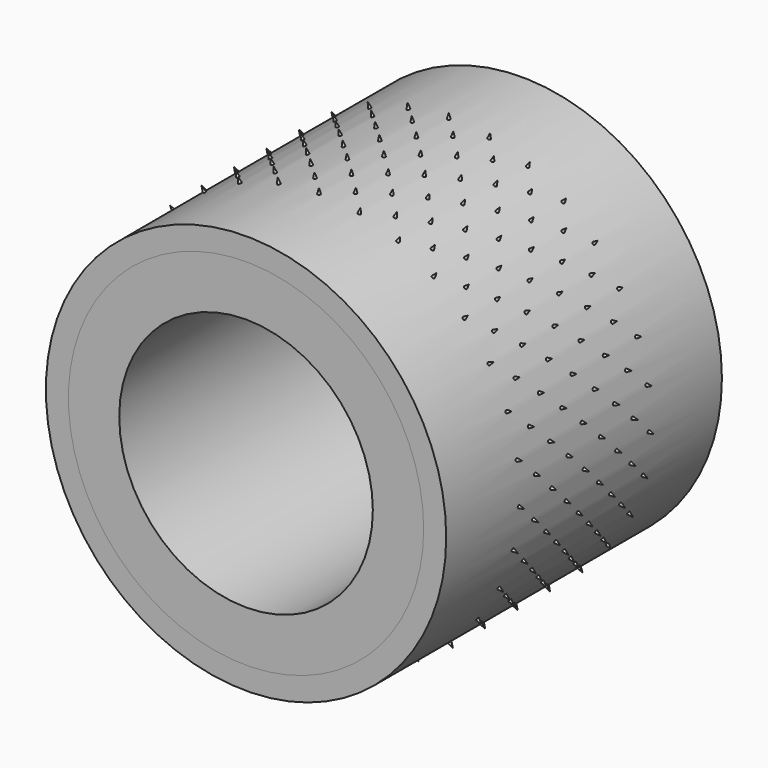
from build123d import *

# Parameters (mm, degrees)
F0_R        = 35.052
F0_R_2      = 25.019
F1_DEPTH    = 34
F2_R        = 39.5
F2_R_2      = 35.052
F3_DEPTH    = 34
F5_R        = 0.31
F6_DEPTH    = 25.4
F8_DEPTH    = 5.5
F9_SIZE2    = 0.31
F9_SIZE     = 1.1
F9_2_SIZE2  = 0.31
F9_2_SIZE   = 1.1
F9_3_SIZE2  = 0.31
F9_3_SIZE   = 1.1
F9_4_SIZE2  = 0.31
F9_4_SIZE   = 1.1
F9_5_SIZE2  = 0.31
F9_5_SIZE   = 1.1
F11_R       = 0.31
F12_DEPTH   = 25.4
F13_DEPTH   = 5.5
F14_SIZE2   = 0.31
F14_SIZE    = 1.1
F14_2_SIZE2 = 0.31
F14_2_SIZE  = 1.1
F14_3_SIZE2 = 0.31
F14_3_SIZE  = 1.1
F14_4_SIZE2 = 0.31
F14_4_SIZE  = 1.1
F15_COUNT   = 31
F15_ANGLE   = 348.387


with BuildPart() as f1:
    # F0 (on Front) → F1 (new body, symmetric)
    with BuildSketch(Plane.XZ):
        Circle(F0_R)
        Circle(F0_R_2, mode=Mode.SUBTRACT)
    extrude(amount=F1_DEPTH, both=True)


with BuildPart() as f3:
    # F2 (on Front) → F3 (new body, symmetric)
    with BuildSketch(Plane.XZ):
        Circle(F2_R)
        Circle(F2_R_2, mode=Mode.SUBTRACT)
    extrude(amount=F3_DEPTH, both=True)

    # F5 (on offset) → F6 (cut)
    with BuildSketch(Plane.XY.offset(35.052)):
        with Locations((0, -16)):
            Circle(F5_R)
        with Locations((0, -8)):
            Circle(F5_R)
        Circle(F5_R)
        with Locations((0, 16)):
            Circle(F5_R)
        with Locations((0, 8)):
            Circle(F5_R)
    extrude(amount=F6_DEPTH, mode=Mode.SUBTRACT)

    # F11 (on offset) → F12 (cut)
    with BuildSketch(Plane.XY.offset(-35.052)):
        with Locations((0, -4)):
            Circle(F11_R)
        with Locations((0, -12)):
            Circle(F11_R)
        with Locations((0, 12)):
            Circle(F11_R)
        with Locations((0, 4)):
            Circle(F11_R)
    extrude(amount=-F12_DEPTH, mode=Mode.SUBTRACT)


with BuildPart() as f8:
    # F5 (on offset) → F8 (new body)
    with BuildSketch(Plane.XY.offset(35.052)):
        with Locations((0, 16)):
            Circle(F5_R)
    extrude(amount=F8_DEPTH)

    # F9
    f9_edges = [f8.edges().sort_by_distance(p)[0] for p in [
        (-0.31, 16, 40.552),
    ]]
    f9_side = f8.faces().sort_by_distance((-0.31, 16, 37.802))[0]
    chamfer(f9_edges, length=F9_SIZE, length2=F9_SIZE2, reference=f9_side)


with BuildPart() as f8b:
    # F5 (on offset) → F8, piece 2 (new body)
    with BuildSketch(Plane.XY.offset(35.052)):
        with Locations((0, 8)):
            Circle(F5_R)
    extrude(amount=F8_DEPTH)

    # F9#2
    f9_2_edges = [f8b.edges().sort_by_distance(p)[0] for p in [
        (-0.31, 8, 40.552),
    ]]
    f9_2_side = f8b.faces().sort_by_distance((-0.31, 8, 37.802))[0]
    chamfer(f9_2_edges, length=F9_2_SIZE, length2=F9_2_SIZE2, reference=f9_2_side)


with BuildPart() as f8c:
    # F5 (on offset) → F8, piece 3 (new body)
    with BuildSketch(Plane.XY.offset(35.052)):
        with Locations((0, -8)):
            Circle(F5_R)
    extrude(amount=F8_DEPTH)

    # F9#3
    f9_3_edges = [f8c.edges().sort_by_distance(p)[0] for p in [
        (-0.31, -8, 40.552),
    ]]
    f9_3_side = f8c.faces().sort_by_distance((-0.31, -8, 37.802))[0]
    chamfer(f9_3_edges, length=F9_3_SIZE, length2=F9_3_SIZE2, reference=f9_3_side)


with BuildPart() as f8d:
    # F5 (on offset) → F8, piece 4 (new body)
    with BuildSketch(Plane.XY.offset(35.052)):
        with Locations((0, -16)):
            Circle(F5_R)
    extrude(amount=F8_DEPTH)

    # F9#4
    f9_4_edges = [f8d.edges().sort_by_distance(p)[0] for p in [
        (-0.31, -16, 40.552),
    ]]
    f9_4_side = f8d.faces().sort_by_distance((-0.31, -16, 37.802))[0]
    chamfer(f9_4_edges, length=F9_4_SIZE, length2=F9_4_SIZE2, reference=f9_4_side)


with BuildPart() as f8e:
    # F5 (on offset) → F8, piece 5 (new body)
    with BuildSketch(Plane.XY.offset(35.052)):
        Circle(F5_R)
    extrude(amount=F8_DEPTH)

    # F9#5
    f9_5_edges = [f8e.edges().sort_by_distance(p)[0] for p in [
        (-0.31, 0, 40.552),
    ]]
    f9_5_side = f8e.faces().sort_by_distance((-0.31, 0, 37.802))[0]
    chamfer(f9_5_edges, length=F9_5_SIZE, length2=F9_5_SIZE2, reference=f9_5_side)


with BuildPart() as f13:
    # F11 (on offset) → F13 (new body)
    with BuildSketch(Plane.XY.offset(-35.052)):
        with Locations((0, -12)):
            Circle(F11_R)
    extrude(amount=-F13_DEPTH)

    # F14
    f14_edges = [f13.edges().sort_by_distance(p)[0] for p in [
        (-0.31, -12, -40.552),
    ]]
    chamfer(f14_edges, length=F14_SIZE, length2=F14_SIZE2)


with BuildPart() as f13b:
    # F11 (on offset) → F13, piece 2 (new body)
    with BuildSketch(Plane.XY.offset(-35.052)):
        with Locations((0, -4)):
            Circle(F11_R)
    extrude(amount=-F13_DEPTH)

    # F14#2
    f14_2_edges = [f13b.edges().sort_by_distance(p)[0] for p in [
        (-0.31, -4, -40.552),
    ]]
    chamfer(f14_2_edges, length=F14_2_SIZE, length2=F14_2_SIZE2)


with BuildPart() as f13c:
    # F11 (on offset) → F13, piece 3 (new body)
    with BuildSketch(Plane.XY.offset(-35.052)):
        with Locations((0, 4)):
            Circle(F11_R)
    extrude(amount=-F13_DEPTH)

    # F14#3
    f14_3_edges = [f13c.edges().sort_by_distance(p)[0] for p in [
        (-0.31, 4, -40.552),
    ]]
    chamfer(f14_3_edges, length=F14_3_SIZE, length2=F14_3_SIZE2)


with BuildPart() as f13d:
    # F11 (on offset) → F13, piece 4 (new body)
    with BuildSketch(Plane.XY.offset(-35.052)):
        with Locations((0, 12)):
            Circle(F11_R)
    extrude(amount=-F13_DEPTH)

    # F14#4
    f14_4_edges = [f13d.edges().sort_by_distance(p)[0] for p in [
        (-0.31, 12, -40.552),
    ]]
    chamfer(f14_4_edges, length=F14_4_SIZE, length2=F14_4_SIZE2)


with BuildPart() as f15_1:
    # F15: instance of F8e
    add(f8e.part.rotate(Axis((0, -2.9214471579, 0), (0, -1, 0)), 1 * F15_ANGLE / (F15_COUNT - 1)))


with BuildPart() as f15_2:
    # F15: instance of F8e
    add(f8e.part.rotate(Axis((0, -2.9214471579, 0), (0, -1, 0)), 2 * F15_ANGLE / (F15_COUNT - 1)))


with BuildPart() as f15_3:
    # F15: instance of F8e
    add(f8e.part.rotate(Axis((0, -2.9214471579, 0), (0, -1, 0)), 3 * F15_ANGLE / (F15_COUNT - 1)))


with BuildPart() as f15_4:
    # F15: instance of F8e
    add(f8e.part.rotate(Axis((0, -2.9214471579, 0), (0, -1, 0)), 4 * F15_ANGLE / (F15_COUNT - 1)))


with BuildPart() as f15_5:
    # F15: instance of F8e
    add(f8e.part.rotate(Axis((0, -2.9214471579, 0), (0, -1, 0)), 5 * F15_ANGLE / (F15_COUNT - 1)))


with BuildPart() as f15_6:
    # F15: instance of F8e
    add(f8e.part.rotate(Axis((0, -2.9214471579, 0), (0, -1, 0)), 6 * F15_ANGLE / (F15_COUNT - 1)))


with BuildPart() as f15_7:
    # F15: instance of F8e
    add(f8e.part.rotate(Axis((0, -2.9214471579, 0), (0, -1, 0)), 7 * F15_ANGLE / (F15_COUNT - 1)))


with BuildPart() as f15_8:
    # F15: instance of F8e
    add(f8e.part.rotate(Axis((0, -2.9214471579, 0), (0, -1, 0)), 8 * F15_ANGLE / (F15_COUNT - 1)))


with BuildPart() as f15_9:
    # F15: instance of F8e
    add(f8e.part.rotate(Axis((0, -2.9214471579, 0), (0, -1, 0)), 9 * F15_ANGLE / (F15_COUNT - 1)))


with BuildPart() as f15_10:
    # F15: instance of F8e
    add(f8e.part.rotate(Axis((0, -2.9214471579, 0), (0, -1, 0)), 10 * F15_ANGLE / (F15_COUNT - 1)))


with BuildPart() as f15_11:
    # F15: instance of F8e
    add(f8e.part.rotate(Axis((0, -2.9214471579, 0), (0, -1, 0)), 11 * F15_ANGLE / (F15_COUNT - 1)))


with BuildPart() as f15_12:
    # F15: instance of F8e
    add(f8e.part.rotate(Axis((0, -2.9214471579, 0), (0, -1, 0)), 12 * F15_ANGLE / (F15_COUNT - 1)))


with BuildPart() as f15_13:
    # F15: instance of F8e
    add(f8e.part.rotate(Axis((0, -2.9214471579, 0), (0, -1, 0)), 13 * F15_ANGLE / (F15_COUNT - 1)))


with BuildPart() as f15_14:
    # F15: instance of F8e
    add(f8e.part.rotate(Axis((0, -2.9214471579, 0), (0, -1, 0)), 14 * F15_ANGLE / (F15_COUNT - 1)))


with BuildPart() as f15_15:
    # F15: instance of F8e
    add(f8e.part.rotate(Axis((0, -2.9214471579, 0), (0, -1, 0)), 15 * F15_ANGLE / (F15_COUNT - 1)))


with BuildPart() as f15_16:
    # F15: instance of F8e
    add(f8e.part.rotate(Axis((0, -2.9214471579, 0), (0, -1, 0)), 16 * F15_ANGLE / (F15_COUNT - 1)))


with BuildPart() as f15_17:
    # F15: instance of F8e
    add(f8e.part.rotate(Axis((0, -2.9214471579, 0), (0, -1, 0)), 17 * F15_ANGLE / (F15_COUNT - 1)))


with BuildPart() as f15_18:
    # F15: instance of F8e
    add(f8e.part.rotate(Axis((0, -2.9214471579, 0), (0, -1, 0)), 18 * F15_ANGLE / (F15_COUNT - 1)))


with BuildPart() as f15_19:
    # F15: instance of F8e
    add(f8e.part.rotate(Axis((0, -2.9214471579, 0), (0, -1, 0)), 19 * F15_ANGLE / (F15_COUNT - 1)))


with BuildPart() as f15_20:
    # F15: instance of F8e
    add(f8e.part.rotate(Axis((0, -2.9214471579, 0), (0, -1, 0)), 20 * F15_ANGLE / (F15_COUNT - 1)))


with BuildPart() as f15_21:
    # F15: instance of F8e
    add(f8e.part.rotate(Axis((0, -2.9214471579, 0), (0, -1, 0)), 21 * F15_ANGLE / (F15_COUNT - 1)))


with BuildPart() as f15_22:
    # F15: instance of F8e
    add(f8e.part.rotate(Axis((0, -2.9214471579, 0), (0, -1, 0)), 22 * F15_ANGLE / (F15_COUNT - 1)))


with BuildPart() as f15_23:
    # F15: instance of F8e
    add(f8e.part.rotate(Axis((0, -2.9214471579, 0), (0, -1, 0)), 23 * F15_ANGLE / (F15_COUNT - 1)))


with BuildPart() as f15_24:
    # F15: instance of F8e
    add(f8e.part.rotate(Axis((0, -2.9214471579, 0), (0, -1, 0)), 24 * F15_ANGLE / (F15_COUNT - 1)))


with BuildPart() as f15_25:
    # F15: instance of F8e
    add(f8e.part.rotate(Axis((0, -2.9214471579, 0), (0, -1, 0)), 25 * F15_ANGLE / (F15_COUNT - 1)))


with BuildPart() as f15_26:
    # F15: instance of F8e
    add(f8e.part.rotate(Axis((0, -2.9214471579, 0), (0, -1, 0)), 26 * F15_ANGLE / (F15_COUNT - 1)))


with BuildPart() as f15_27:
    # F15: instance of F8e
    add(f8e.part.rotate(Axis((0, -2.9214471579, 0), (0, -1, 0)), 27 * F15_ANGLE / (F15_COUNT - 1)))


with BuildPart() as f15_28:
    # F15: instance of F8e
    add(f8e.part.rotate(Axis((0, -2.9214471579, 0), (0, -1, 0)), 28 * F15_ANGLE / (F15_COUNT - 1)))


with BuildPart() as f15_29:
    # F15: instance of F8e
    add(f8e.part.rotate(Axis((0, -2.9214471579, 0), (0, -1, 0)), 29 * F15_ANGLE / (F15_COUNT - 1)))


with BuildPart() as f15_30:
    # F15: instance of F8e
    add(f8e.part.rotate(Axis((0, -2.9214471579, 0), (0, -1, 0)), 30 * F15_ANGLE / (F15_COUNT - 1)))


with BuildPart() as f15_31:
    # F15: instance of F8b
    add(f8b.part.rotate(Axis((0, -2.9214471579, 0), (0, -1, 0)), 1 * F15_ANGLE / (F15_COUNT - 1)))


with BuildPart() as f15_32:
    # F15: instance of F8b
    add(f8b.part.rotate(Axis((0, -2.9214471579, 0), (0, -1, 0)), 2 * F15_ANGLE / (F15_COUNT - 1)))


with BuildPart() as f15_33:
    # F15: instance of F8b
    add(f8b.part.rotate(Axis((0, -2.9214471579, 0), (0, -1, 0)), 3 * F15_ANGLE / (F15_COUNT - 1)))


with BuildPart() as f15_34:
    # F15: instance of F8b
    add(f8b.part.rotate(Axis((0, -2.9214471579, 0), (0, -1, 0)), 4 * F15_ANGLE / (F15_COUNT - 1)))


with BuildPart() as f15_35:
    # F15: instance of F8b
    add(f8b.part.rotate(Axis((0, -2.9214471579, 0), (0, -1, 0)), 5 * F15_ANGLE / (F15_COUNT - 1)))


with BuildPart() as f15_36:
    # F15: instance of F8b
    add(f8b.part.rotate(Axis((0, -2.9214471579, 0), (0, -1, 0)), 6 * F15_ANGLE / (F15_COUNT - 1)))


with BuildPart() as f15_37:
    # F15: instance of F8b
    add(f8b.part.rotate(Axis((0, -2.9214471579, 0), (0, -1, 0)), 7 * F15_ANGLE / (F15_COUNT - 1)))


with BuildPart() as f15_38:
    # F15: instance of F8b
    add(f8b.part.rotate(Axis((0, -2.9214471579, 0), (0, -1, 0)), 8 * F15_ANGLE / (F15_COUNT - 1)))


with BuildPart() as f15_39:
    # F15: instance of F8b
    add(f8b.part.rotate(Axis((0, -2.9214471579, 0), (0, -1, 0)), 9 * F15_ANGLE / (F15_COUNT - 1)))


with BuildPart() as f15_40:
    # F15: instance of F8b
    add(f8b.part.rotate(Axis((0, -2.9214471579, 0), (0, -1, 0)), 10 * F15_ANGLE / (F15_COUNT - 1)))


with BuildPart() as f15_41:
    # F15: instance of F8b
    add(f8b.part.rotate(Axis((0, -2.9214471579, 0), (0, -1, 0)), 11 * F15_ANGLE / (F15_COUNT - 1)))


with BuildPart() as f15_42:
    # F15: instance of F8b
    add(f8b.part.rotate(Axis((0, -2.9214471579, 0), (0, -1, 0)), 12 * F15_ANGLE / (F15_COUNT - 1)))


with BuildPart() as f15_43:
    # F15: instance of F8b
    add(f8b.part.rotate(Axis((0, -2.9214471579, 0), (0, -1, 0)), 13 * F15_ANGLE / (F15_COUNT - 1)))


with BuildPart() as f15_44:
    # F15: instance of F8b
    add(f8b.part.rotate(Axis((0, -2.9214471579, 0), (0, -1, 0)), 14 * F15_ANGLE / (F15_COUNT - 1)))


with BuildPart() as f15_45:
    # F15: instance of F8b
    add(f8b.part.rotate(Axis((0, -2.9214471579, 0), (0, -1, 0)), 15 * F15_ANGLE / (F15_COUNT - 1)))


with BuildPart() as f15_46:
    # F15: instance of F8b
    add(f8b.part.rotate(Axis((0, -2.9214471579, 0), (0, -1, 0)), 16 * F15_ANGLE / (F15_COUNT - 1)))


with BuildPart() as f15_47:
    # F15: instance of F8b
    add(f8b.part.rotate(Axis((0, -2.9214471579, 0), (0, -1, 0)), 17 * F15_ANGLE / (F15_COUNT - 1)))


with BuildPart() as f15_48:
    # F15: instance of F8b
    add(f8b.part.rotate(Axis((0, -2.9214471579, 0), (0, -1, 0)), 18 * F15_ANGLE / (F15_COUNT - 1)))


with BuildPart() as f15_49:
    # F15: instance of F8b
    add(f8b.part.rotate(Axis((0, -2.9214471579, 0), (0, -1, 0)), 19 * F15_ANGLE / (F15_COUNT - 1)))


with BuildPart() as f15_50:
    # F15: instance of F8b
    add(f8b.part.rotate(Axis((0, -2.9214471579, 0), (0, -1, 0)), 20 * F15_ANGLE / (F15_COUNT - 1)))


with BuildPart() as f15_51:
    # F15: instance of F8b
    add(f8b.part.rotate(Axis((0, -2.9214471579, 0), (0, -1, 0)), 21 * F15_ANGLE / (F15_COUNT - 1)))


with BuildPart() as f15_52:
    # F15: instance of F8b
    add(f8b.part.rotate(Axis((0, -2.9214471579, 0), (0, -1, 0)), 22 * F15_ANGLE / (F15_COUNT - 1)))


with BuildPart() as f15_53:
    # F15: instance of F8b
    add(f8b.part.rotate(Axis((0, -2.9214471579, 0), (0, -1, 0)), 23 * F15_ANGLE / (F15_COUNT - 1)))


with BuildPart() as f15_54:
    # F15: instance of F8b
    add(f8b.part.rotate(Axis((0, -2.9214471579, 0), (0, -1, 0)), 24 * F15_ANGLE / (F15_COUNT - 1)))


with BuildPart() as f15_55:
    # F15: instance of F8b
    add(f8b.part.rotate(Axis((0, -2.9214471579, 0), (0, -1, 0)), 25 * F15_ANGLE / (F15_COUNT - 1)))


with BuildPart() as f15_56:
    # F15: instance of F8b
    add(f8b.part.rotate(Axis((0, -2.9214471579, 0), (0, -1, 0)), 26 * F15_ANGLE / (F15_COUNT - 1)))


with BuildPart() as f15_57:
    # F15: instance of F8b
    add(f8b.part.rotate(Axis((0, -2.9214471579, 0), (0, -1, 0)), 27 * F15_ANGLE / (F15_COUNT - 1)))


with BuildPart() as f15_58:
    # F15: instance of F8b
    add(f8b.part.rotate(Axis((0, -2.9214471579, 0), (0, -1, 0)), 28 * F15_ANGLE / (F15_COUNT - 1)))


with BuildPart() as f15_59:
    # F15: instance of F8b
    add(f8b.part.rotate(Axis((0, -2.9214471579, 0), (0, -1, 0)), 29 * F15_ANGLE / (F15_COUNT - 1)))


with BuildPart() as f15_60:
    # F15: instance of F8b
    add(f8b.part.rotate(Axis((0, -2.9214471579, 0), (0, -1, 0)), 30 * F15_ANGLE / (F15_COUNT - 1)))


with BuildPart() as f15_61:
    # F15: instance of F8
    add(f8.part.rotate(Axis((0, -2.9214471579, 0), (0, -1, 0)), 1 * F15_ANGLE / (F15_COUNT - 1)))


with BuildPart() as f15_62:
    # F15: instance of F8
    add(f8.part.rotate(Axis((0, -2.9214471579, 0), (0, -1, 0)), 2 * F15_ANGLE / (F15_COUNT - 1)))


with BuildPart() as f15_63:
    # F15: instance of F8
    add(f8.part.rotate(Axis((0, -2.9214471579, 0), (0, -1, 0)), 3 * F15_ANGLE / (F15_COUNT - 1)))


with BuildPart() as f15_64:
    # F15: instance of F8
    add(f8.part.rotate(Axis((0, -2.9214471579, 0), (0, -1, 0)), 4 * F15_ANGLE / (F15_COUNT - 1)))


with BuildPart() as f15_65:
    # F15: instance of F8
    add(f8.part.rotate(Axis((0, -2.9214471579, 0), (0, -1, 0)), 5 * F15_ANGLE / (F15_COUNT - 1)))


with BuildPart() as f15_66:
    # F15: instance of F8
    add(f8.part.rotate(Axis((0, -2.9214471579, 0), (0, -1, 0)), 6 * F15_ANGLE / (F15_COUNT - 1)))


with BuildPart() as f15_67:
    # F15: instance of F8
    add(f8.part.rotate(Axis((0, -2.9214471579, 0), (0, -1, 0)), 7 * F15_ANGLE / (F15_COUNT - 1)))


with BuildPart() as f15_68:
    # F15: instance of F8
    add(f8.part.rotate(Axis((0, -2.9214471579, 0), (0, -1, 0)), 8 * F15_ANGLE / (F15_COUNT - 1)))


with BuildPart() as f15_69:
    # F15: instance of F8
    add(f8.part.rotate(Axis((0, -2.9214471579, 0), (0, -1, 0)), 9 * F15_ANGLE / (F15_COUNT - 1)))


with BuildPart() as f15_70:
    # F15: instance of F8
    add(f8.part.rotate(Axis((0, -2.9214471579, 0), (0, -1, 0)), 10 * F15_ANGLE / (F15_COUNT - 1)))


with BuildPart() as f15_71:
    # F15: instance of F8
    add(f8.part.rotate(Axis((0, -2.9214471579, 0), (0, -1, 0)), 11 * F15_ANGLE / (F15_COUNT - 1)))


with BuildPart() as f15_72:
    # F15: instance of F8
    add(f8.part.rotate(Axis((0, -2.9214471579, 0), (0, -1, 0)), 12 * F15_ANGLE / (F15_COUNT - 1)))


with BuildPart() as f15_73:
    # F15: instance of F8
    add(f8.part.rotate(Axis((0, -2.9214471579, 0), (0, -1, 0)), 13 * F15_ANGLE / (F15_COUNT - 1)))


with BuildPart() as f15_74:
    # F15: instance of F8
    add(f8.part.rotate(Axis((0, -2.9214471579, 0), (0, -1, 0)), 14 * F15_ANGLE / (F15_COUNT - 1)))


with BuildPart() as f15_75:
    # F15: instance of F8
    add(f8.part.rotate(Axis((0, -2.9214471579, 0), (0, -1, 0)), 15 * F15_ANGLE / (F15_COUNT - 1)))


with BuildPart() as f15_76:
    # F15: instance of F8
    add(f8.part.rotate(Axis((0, -2.9214471579, 0), (0, -1, 0)), 16 * F15_ANGLE / (F15_COUNT - 1)))


with BuildPart() as f15_77:
    # F15: instance of F8
    add(f8.part.rotate(Axis((0, -2.9214471579, 0), (0, -1, 0)), 17 * F15_ANGLE / (F15_COUNT - 1)))


with BuildPart() as f15_78:
    # F15: instance of F8
    add(f8.part.rotate(Axis((0, -2.9214471579, 0), (0, -1, 0)), 18 * F15_ANGLE / (F15_COUNT - 1)))


with BuildPart() as f15_79:
    # F15: instance of F8
    add(f8.part.rotate(Axis((0, -2.9214471579, 0), (0, -1, 0)), 19 * F15_ANGLE / (F15_COUNT - 1)))


with BuildPart() as f15_80:
    # F15: instance of F8
    add(f8.part.rotate(Axis((0, -2.9214471579, 0), (0, -1, 0)), 20 * F15_ANGLE / (F15_COUNT - 1)))


with BuildPart() as f15_81:
    # F15: instance of F8
    add(f8.part.rotate(Axis((0, -2.9214471579, 0), (0, -1, 0)), 21 * F15_ANGLE / (F15_COUNT - 1)))


with BuildPart() as f15_82:
    # F15: instance of F8
    add(f8.part.rotate(Axis((0, -2.9214471579, 0), (0, -1, 0)), 22 * F15_ANGLE / (F15_COUNT - 1)))


with BuildPart() as f15_83:
    # F15: instance of F8
    add(f8.part.rotate(Axis((0, -2.9214471579, 0), (0, -1, 0)), 23 * F15_ANGLE / (F15_COUNT - 1)))


with BuildPart() as f15_84:
    # F15: instance of F8
    add(f8.part.rotate(Axis((0, -2.9214471579, 0), (0, -1, 0)), 24 * F15_ANGLE / (F15_COUNT - 1)))


with BuildPart() as f15_85:
    # F15: instance of F8
    add(f8.part.rotate(Axis((0, -2.9214471579, 0), (0, -1, 0)), 25 * F15_ANGLE / (F15_COUNT - 1)))


with BuildPart() as f15_86:
    # F15: instance of F8
    add(f8.part.rotate(Axis((0, -2.9214471579, 0), (0, -1, 0)), 26 * F15_ANGLE / (F15_COUNT - 1)))


with BuildPart() as f15_87:
    # F15: instance of F8
    add(f8.part.rotate(Axis((0, -2.9214471579, 0), (0, -1, 0)), 27 * F15_ANGLE / (F15_COUNT - 1)))


with BuildPart() as f15_88:
    # F15: instance of F8
    add(f8.part.rotate(Axis((0, -2.9214471579, 0), (0, -1, 0)), 28 * F15_ANGLE / (F15_COUNT - 1)))


with BuildPart() as f15_89:
    # F15: instance of F8
    add(f8.part.rotate(Axis((0, -2.9214471579, 0), (0, -1, 0)), 29 * F15_ANGLE / (F15_COUNT - 1)))


with BuildPart() as f15_90:
    # F15: instance of F8
    add(f8.part.rotate(Axis((0, -2.9214471579, 0), (0, -1, 0)), 30 * F15_ANGLE / (F15_COUNT - 1)))


with BuildPart() as f15_91:
    # F15: instance of F8c
    add(f8c.part.rotate(Axis((0, -2.9214471579, 0), (0, -1, 0)), 1 * F15_ANGLE / (F15_COUNT - 1)))


with BuildPart() as f15_92:
    # F15: instance of F8c
    add(f8c.part.rotate(Axis((0, -2.9214471579, 0), (0, -1, 0)), 2 * F15_ANGLE / (F15_COUNT - 1)))


with BuildPart() as f15_93:
    # F15: instance of F8c
    add(f8c.part.rotate(Axis((0, -2.9214471579, 0), (0, -1, 0)), 3 * F15_ANGLE / (F15_COUNT - 1)))


with BuildPart() as f15_94:
    # F15: instance of F8c
    add(f8c.part.rotate(Axis((0, -2.9214471579, 0), (0, -1, 0)), 4 * F15_ANGLE / (F15_COUNT - 1)))


with BuildPart() as f15_95:
    # F15: instance of F8c
    add(f8c.part.rotate(Axis((0, -2.9214471579, 0), (0, -1, 0)), 5 * F15_ANGLE / (F15_COUNT - 1)))


with BuildPart() as f15_96:
    # F15: instance of F8c
    add(f8c.part.rotate(Axis((0, -2.9214471579, 0), (0, -1, 0)), 6 * F15_ANGLE / (F15_COUNT - 1)))


with BuildPart() as f15_97:
    # F15: instance of F8c
    add(f8c.part.rotate(Axis((0, -2.9214471579, 0), (0, -1, 0)), 7 * F15_ANGLE / (F15_COUNT - 1)))


with BuildPart() as f15_98:
    # F15: instance of F8c
    add(f8c.part.rotate(Axis((0, -2.9214471579, 0), (0, -1, 0)), 8 * F15_ANGLE / (F15_COUNT - 1)))


with BuildPart() as f15_99:
    # F15: instance of F8c
    add(f8c.part.rotate(Axis((0, -2.9214471579, 0), (0, -1, 0)), 9 * F15_ANGLE / (F15_COUNT - 1)))


with BuildPart() as f15_100:
    # F15: instance of F8c
    add(f8c.part.rotate(Axis((0, -2.9214471579, 0), (0, -1, 0)), 10 * F15_ANGLE / (F15_COUNT - 1)))


with BuildPart() as f15_101:
    # F15: instance of F8c
    add(f8c.part.rotate(Axis((0, -2.9214471579, 0), (0, -1, 0)), 11 * F15_ANGLE / (F15_COUNT - 1)))


with BuildPart() as f15_102:
    # F15: instance of F8c
    add(f8c.part.rotate(Axis((0, -2.9214471579, 0), (0, -1, 0)), 12 * F15_ANGLE / (F15_COUNT - 1)))


with BuildPart() as f15_103:
    # F15: instance of F8c
    add(f8c.part.rotate(Axis((0, -2.9214471579, 0), (0, -1, 0)), 13 * F15_ANGLE / (F15_COUNT - 1)))


with BuildPart() as f15_104:
    # F15: instance of F8c
    add(f8c.part.rotate(Axis((0, -2.9214471579, 0), (0, -1, 0)), 14 * F15_ANGLE / (F15_COUNT - 1)))


with BuildPart() as f15_105:
    # F15: instance of F8c
    add(f8c.part.rotate(Axis((0, -2.9214471579, 0), (0, -1, 0)), 15 * F15_ANGLE / (F15_COUNT - 1)))


with BuildPart() as f15_106:
    # F15: instance of F8c
    add(f8c.part.rotate(Axis((0, -2.9214471579, 0), (0, -1, 0)), 16 * F15_ANGLE / (F15_COUNT - 1)))


with BuildPart() as f15_107:
    # F15: instance of F8c
    add(f8c.part.rotate(Axis((0, -2.9214471579, 0), (0, -1, 0)), 17 * F15_ANGLE / (F15_COUNT - 1)))


with BuildPart() as f15_108:
    # F15: instance of F8c
    add(f8c.part.rotate(Axis((0, -2.9214471579, 0), (0, -1, 0)), 18 * F15_ANGLE / (F15_COUNT - 1)))


with BuildPart() as f15_109:
    # F15: instance of F8c
    add(f8c.part.rotate(Axis((0, -2.9214471579, 0), (0, -1, 0)), 19 * F15_ANGLE / (F15_COUNT - 1)))


with BuildPart() as f15_110:
    # F15: instance of F8c
    add(f8c.part.rotate(Axis((0, -2.9214471579, 0), (0, -1, 0)), 20 * F15_ANGLE / (F15_COUNT - 1)))


with BuildPart() as f15_111:
    # F15: instance of F8c
    add(f8c.part.rotate(Axis((0, -2.9214471579, 0), (0, -1, 0)), 21 * F15_ANGLE / (F15_COUNT - 1)))


with BuildPart() as f15_112:
    # F15: instance of F8c
    add(f8c.part.rotate(Axis((0, -2.9214471579, 0), (0, -1, 0)), 22 * F15_ANGLE / (F15_COUNT - 1)))


with BuildPart() as f15_113:
    # F15: instance of F8c
    add(f8c.part.rotate(Axis((0, -2.9214471579, 0), (0, -1, 0)), 23 * F15_ANGLE / (F15_COUNT - 1)))


with BuildPart() as f15_114:
    # F15: instance of F8c
    add(f8c.part.rotate(Axis((0, -2.9214471579, 0), (0, -1, 0)), 24 * F15_ANGLE / (F15_COUNT - 1)))


with BuildPart() as f15_115:
    # F15: instance of F8c
    add(f8c.part.rotate(Axis((0, -2.9214471579, 0), (0, -1, 0)), 25 * F15_ANGLE / (F15_COUNT - 1)))


with BuildPart() as f15_116:
    # F15: instance of F8c
    add(f8c.part.rotate(Axis((0, -2.9214471579, 0), (0, -1, 0)), 26 * F15_ANGLE / (F15_COUNT - 1)))


with BuildPart() as f15_117:
    # F15: instance of F8c
    add(f8c.part.rotate(Axis((0, -2.9214471579, 0), (0, -1, 0)), 27 * F15_ANGLE / (F15_COUNT - 1)))


with BuildPart() as f15_118:
    # F15: instance of F8c
    add(f8c.part.rotate(Axis((0, -2.9214471579, 0), (0, -1, 0)), 28 * F15_ANGLE / (F15_COUNT - 1)))


with BuildPart() as f15_119:
    # F15: instance of F8c
    add(f8c.part.rotate(Axis((0, -2.9214471579, 0), (0, -1, 0)), 29 * F15_ANGLE / (F15_COUNT - 1)))


with BuildPart() as f15_120:
    # F15: instance of F8c
    add(f8c.part.rotate(Axis((0, -2.9214471579, 0), (0, -1, 0)), 30 * F15_ANGLE / (F15_COUNT - 1)))


with BuildPart() as f15_121:
    # F15: instance of F8d
    add(f8d.part.rotate(Axis((0, -2.9214471579, 0), (0, -1, 0)), 1 * F15_ANGLE / (F15_COUNT - 1)))


with BuildPart() as f15_122:
    # F15: instance of F8d
    add(f8d.part.rotate(Axis((0, -2.9214471579, 0), (0, -1, 0)), 2 * F15_ANGLE / (F15_COUNT - 1)))


with BuildPart() as f15_123:
    # F15: instance of F8d
    add(f8d.part.rotate(Axis((0, -2.9214471579, 0), (0, -1, 0)), 3 * F15_ANGLE / (F15_COUNT - 1)))


with BuildPart() as f15_124:
    # F15: instance of F8d
    add(f8d.part.rotate(Axis((0, -2.9214471579, 0), (0, -1, 0)), 4 * F15_ANGLE / (F15_COUNT - 1)))


with BuildPart() as f15_125:
    # F15: instance of F8d
    add(f8d.part.rotate(Axis((0, -2.9214471579, 0), (0, -1, 0)), 5 * F15_ANGLE / (F15_COUNT - 1)))


with BuildPart() as f15_126:
    # F15: instance of F8d
    add(f8d.part.rotate(Axis((0, -2.9214471579, 0), (0, -1, 0)), 6 * F15_ANGLE / (F15_COUNT - 1)))


with BuildPart() as f15_127:
    # F15: instance of F8d
    add(f8d.part.rotate(Axis((0, -2.9214471579, 0), (0, -1, 0)), 7 * F15_ANGLE / (F15_COUNT - 1)))


with BuildPart() as f15_128:
    # F15: instance of F8d
    add(f8d.part.rotate(Axis((0, -2.9214471579, 0), (0, -1, 0)), 8 * F15_ANGLE / (F15_COUNT - 1)))


with BuildPart() as f15_129:
    # F15: instance of F8d
    add(f8d.part.rotate(Axis((0, -2.9214471579, 0), (0, -1, 0)), 9 * F15_ANGLE / (F15_COUNT - 1)))


with BuildPart() as f15_130:
    # F15: instance of F8d
    add(f8d.part.rotate(Axis((0, -2.9214471579, 0), (0, -1, 0)), 10 * F15_ANGLE / (F15_COUNT - 1)))


with BuildPart() as f15_131:
    # F15: instance of F8d
    add(f8d.part.rotate(Axis((0, -2.9214471579, 0), (0, -1, 0)), 11 * F15_ANGLE / (F15_COUNT - 1)))


with BuildPart() as f15_132:
    # F15: instance of F8d
    add(f8d.part.rotate(Axis((0, -2.9214471579, 0), (0, -1, 0)), 12 * F15_ANGLE / (F15_COUNT - 1)))


with BuildPart() as f15_133:
    # F15: instance of F8d
    add(f8d.part.rotate(Axis((0, -2.9214471579, 0), (0, -1, 0)), 13 * F15_ANGLE / (F15_COUNT - 1)))


with BuildPart() as f15_134:
    # F15: instance of F8d
    add(f8d.part.rotate(Axis((0, -2.9214471579, 0), (0, -1, 0)), 14 * F15_ANGLE / (F15_COUNT - 1)))


with BuildPart() as f15_135:
    # F15: instance of F8d
    add(f8d.part.rotate(Axis((0, -2.9214471579, 0), (0, -1, 0)), 15 * F15_ANGLE / (F15_COUNT - 1)))


with BuildPart() as f15_136:
    # F15: instance of F8d
    add(f8d.part.rotate(Axis((0, -2.9214471579, 0), (0, -1, 0)), 16 * F15_ANGLE / (F15_COUNT - 1)))


with BuildPart() as f15_137:
    # F15: instance of F8d
    add(f8d.part.rotate(Axis((0, -2.9214471579, 0), (0, -1, 0)), 17 * F15_ANGLE / (F15_COUNT - 1)))


with BuildPart() as f15_138:
    # F15: instance of F8d
    add(f8d.part.rotate(Axis((0, -2.9214471579, 0), (0, -1, 0)), 18 * F15_ANGLE / (F15_COUNT - 1)))


with BuildPart() as f15_139:
    # F15: instance of F8d
    add(f8d.part.rotate(Axis((0, -2.9214471579, 0), (0, -1, 0)), 19 * F15_ANGLE / (F15_COUNT - 1)))


with BuildPart() as f15_140:
    # F15: instance of F8d
    add(f8d.part.rotate(Axis((0, -2.9214471579, 0), (0, -1, 0)), 20 * F15_ANGLE / (F15_COUNT - 1)))


with BuildPart() as f15_141:
    # F15: instance of F8d
    add(f8d.part.rotate(Axis((0, -2.9214471579, 0), (0, -1, 0)), 21 * F15_ANGLE / (F15_COUNT - 1)))


with BuildPart() as f15_142:
    # F15: instance of F8d
    add(f8d.part.rotate(Axis((0, -2.9214471579, 0), (0, -1, 0)), 22 * F15_ANGLE / (F15_COUNT - 1)))


with BuildPart() as f15_143:
    # F15: instance of F8d
    add(f8d.part.rotate(Axis((0, -2.9214471579, 0), (0, -1, 0)), 23 * F15_ANGLE / (F15_COUNT - 1)))


with BuildPart() as f15_144:
    # F15: instance of F8d
    add(f8d.part.rotate(Axis((0, -2.9214471579, 0), (0, -1, 0)), 24 * F15_ANGLE / (F15_COUNT - 1)))


with BuildPart() as f15_145:
    # F15: instance of F8d
    add(f8d.part.rotate(Axis((0, -2.9214471579, 0), (0, -1, 0)), 25 * F15_ANGLE / (F15_COUNT - 1)))


with BuildPart() as f15_146:
    # F15: instance of F8d
    add(f8d.part.rotate(Axis((0, -2.9214471579, 0), (0, -1, 0)), 26 * F15_ANGLE / (F15_COUNT - 1)))


with BuildPart() as f15_147:
    # F15: instance of F8d
    add(f8d.part.rotate(Axis((0, -2.9214471579, 0), (0, -1, 0)), 27 * F15_ANGLE / (F15_COUNT - 1)))


with BuildPart() as f15_148:
    # F15: instance of F8d
    add(f8d.part.rotate(Axis((0, -2.9214471579, 0), (0, -1, 0)), 28 * F15_ANGLE / (F15_COUNT - 1)))


with BuildPart() as f15_149:
    # F15: instance of F8d
    add(f8d.part.rotate(Axis((0, -2.9214471579, 0), (0, -1, 0)), 29 * F15_ANGLE / (F15_COUNT - 1)))


with BuildPart() as f15_150:
    # F15: instance of F8d
    add(f8d.part.rotate(Axis((0, -2.9214471579, 0), (0, -1, 0)), 30 * F15_ANGLE / (F15_COUNT - 1)))


with BuildPart() as f15_151:
    # F15: instance of F13b
    add(f13b.part.rotate(Axis((0, -2.9214471579, 0), (0, -1, 0)), 1 * F15_ANGLE / (F15_COUNT - 1)))


with BuildPart() as f15_152:
    # F15: instance of F13b
    add(f13b.part.rotate(Axis((0, -2.9214471579, 0), (0, -1, 0)), 2 * F15_ANGLE / (F15_COUNT - 1)))


with BuildPart() as f15_153:
    # F15: instance of F13b
    add(f13b.part.rotate(Axis((0, -2.9214471579, 0), (0, -1, 0)), 3 * F15_ANGLE / (F15_COUNT - 1)))


with BuildPart() as f15_154:
    # F15: instance of F13b
    add(f13b.part.rotate(Axis((0, -2.9214471579, 0), (0, -1, 0)), 4 * F15_ANGLE / (F15_COUNT - 1)))


with BuildPart() as f15_155:
    # F15: instance of F13b
    add(f13b.part.rotate(Axis((0, -2.9214471579, 0), (0, -1, 0)), 5 * F15_ANGLE / (F15_COUNT - 1)))


with BuildPart() as f15_156:
    # F15: instance of F13b
    add(f13b.part.rotate(Axis((0, -2.9214471579, 0), (0, -1, 0)), 6 * F15_ANGLE / (F15_COUNT - 1)))


with BuildPart() as f15_157:
    # F15: instance of F13b
    add(f13b.part.rotate(Axis((0, -2.9214471579, 0), (0, -1, 0)), 7 * F15_ANGLE / (F15_COUNT - 1)))


with BuildPart() as f15_158:
    # F15: instance of F13b
    add(f13b.part.rotate(Axis((0, -2.9214471579, 0), (0, -1, 0)), 8 * F15_ANGLE / (F15_COUNT - 1)))


with BuildPart() as f15_159:
    # F15: instance of F13b
    add(f13b.part.rotate(Axis((0, -2.9214471579, 0), (0, -1, 0)), 9 * F15_ANGLE / (F15_COUNT - 1)))


with BuildPart() as f15_160:
    # F15: instance of F13b
    add(f13b.part.rotate(Axis((0, -2.9214471579, 0), (0, -1, 0)), 10 * F15_ANGLE / (F15_COUNT - 1)))


with BuildPart() as f15_161:
    # F15: instance of F13b
    add(f13b.part.rotate(Axis((0, -2.9214471579, 0), (0, -1, 0)), 11 * F15_ANGLE / (F15_COUNT - 1)))


with BuildPart() as f15_162:
    # F15: instance of F13b
    add(f13b.part.rotate(Axis((0, -2.9214471579, 0), (0, -1, 0)), 12 * F15_ANGLE / (F15_COUNT - 1)))


with BuildPart() as f15_163:
    # F15: instance of F13b
    add(f13b.part.rotate(Axis((0, -2.9214471579, 0), (0, -1, 0)), 13 * F15_ANGLE / (F15_COUNT - 1)))


with BuildPart() as f15_164:
    # F15: instance of F13b
    add(f13b.part.rotate(Axis((0, -2.9214471579, 0), (0, -1, 0)), 14 * F15_ANGLE / (F15_COUNT - 1)))


with BuildPart() as f15_165:
    # F15: instance of F13b
    add(f13b.part.rotate(Axis((0, -2.9214471579, 0), (0, -1, 0)), 15 * F15_ANGLE / (F15_COUNT - 1)))


with BuildPart() as f15_166:
    # F15: instance of F13b
    add(f13b.part.rotate(Axis((0, -2.9214471579, 0), (0, -1, 0)), 16 * F15_ANGLE / (F15_COUNT - 1)))


with BuildPart() as f15_167:
    # F15: instance of F13b
    add(f13b.part.rotate(Axis((0, -2.9214471579, 0), (0, -1, 0)), 17 * F15_ANGLE / (F15_COUNT - 1)))


with BuildPart() as f15_168:
    # F15: instance of F13b
    add(f13b.part.rotate(Axis((0, -2.9214471579, 0), (0, -1, 0)), 18 * F15_ANGLE / (F15_COUNT - 1)))


with BuildPart() as f15_169:
    # F15: instance of F13b
    add(f13b.part.rotate(Axis((0, -2.9214471579, 0), (0, -1, 0)), 19 * F15_ANGLE / (F15_COUNT - 1)))


with BuildPart() as f15_170:
    # F15: instance of F13b
    add(f13b.part.rotate(Axis((0, -2.9214471579, 0), (0, -1, 0)), 20 * F15_ANGLE / (F15_COUNT - 1)))


with BuildPart() as f15_171:
    # F15: instance of F13b
    add(f13b.part.rotate(Axis((0, -2.9214471579, 0), (0, -1, 0)), 21 * F15_ANGLE / (F15_COUNT - 1)))


with BuildPart() as f15_172:
    # F15: instance of F13b
    add(f13b.part.rotate(Axis((0, -2.9214471579, 0), (0, -1, 0)), 22 * F15_ANGLE / (F15_COUNT - 1)))


with BuildPart() as f15_173:
    # F15: instance of F13b
    add(f13b.part.rotate(Axis((0, -2.9214471579, 0), (0, -1, 0)), 23 * F15_ANGLE / (F15_COUNT - 1)))


with BuildPart() as f15_174:
    # F15: instance of F13b
    add(f13b.part.rotate(Axis((0, -2.9214471579, 0), (0, -1, 0)), 24 * F15_ANGLE / (F15_COUNT - 1)))


with BuildPart() as f15_175:
    # F15: instance of F13b
    add(f13b.part.rotate(Axis((0, -2.9214471579, 0), (0, -1, 0)), 25 * F15_ANGLE / (F15_COUNT - 1)))


with BuildPart() as f15_176:
    # F15: instance of F13b
    add(f13b.part.rotate(Axis((0, -2.9214471579, 0), (0, -1, 0)), 26 * F15_ANGLE / (F15_COUNT - 1)))


with BuildPart() as f15_177:
    # F15: instance of F13b
    add(f13b.part.rotate(Axis((0, -2.9214471579, 0), (0, -1, 0)), 27 * F15_ANGLE / (F15_COUNT - 1)))


with BuildPart() as f15_178:
    # F15: instance of F13b
    add(f13b.part.rotate(Axis((0, -2.9214471579, 0), (0, -1, 0)), 28 * F15_ANGLE / (F15_COUNT - 1)))


with BuildPart() as f15_179:
    # F15: instance of F13b
    add(f13b.part.rotate(Axis((0, -2.9214471579, 0), (0, -1, 0)), 29 * F15_ANGLE / (F15_COUNT - 1)))


with BuildPart() as f15_180:
    # F15: instance of F13b
    add(f13b.part.rotate(Axis((0, -2.9214471579, 0), (0, -1, 0)), 30 * F15_ANGLE / (F15_COUNT - 1)))


with BuildPart() as f15_181:
    # F15: instance of F13c
    add(f13c.part.rotate(Axis((0, -2.9214471579, 0), (0, -1, 0)), 1 * F15_ANGLE / (F15_COUNT - 1)))


with BuildPart() as f15_182:
    # F15: instance of F13c
    add(f13c.part.rotate(Axis((0, -2.9214471579, 0), (0, -1, 0)), 2 * F15_ANGLE / (F15_COUNT - 1)))


with BuildPart() as f15_183:
    # F15: instance of F13c
    add(f13c.part.rotate(Axis((0, -2.9214471579, 0), (0, -1, 0)), 3 * F15_ANGLE / (F15_COUNT - 1)))


with BuildPart() as f15_184:
    # F15: instance of F13c
    add(f13c.part.rotate(Axis((0, -2.9214471579, 0), (0, -1, 0)), 4 * F15_ANGLE / (F15_COUNT - 1)))


with BuildPart() as f15_185:
    # F15: instance of F13c
    add(f13c.part.rotate(Axis((0, -2.9214471579, 0), (0, -1, 0)), 5 * F15_ANGLE / (F15_COUNT - 1)))


with BuildPart() as f15_186:
    # F15: instance of F13c
    add(f13c.part.rotate(Axis((0, -2.9214471579, 0), (0, -1, 0)), 6 * F15_ANGLE / (F15_COUNT - 1)))


with BuildPart() as f15_187:
    # F15: instance of F13c
    add(f13c.part.rotate(Axis((0, -2.9214471579, 0), (0, -1, 0)), 7 * F15_ANGLE / (F15_COUNT - 1)))


with BuildPart() as f15_188:
    # F15: instance of F13c
    add(f13c.part.rotate(Axis((0, -2.9214471579, 0), (0, -1, 0)), 8 * F15_ANGLE / (F15_COUNT - 1)))


with BuildPart() as f15_189:
    # F15: instance of F13c
    add(f13c.part.rotate(Axis((0, -2.9214471579, 0), (0, -1, 0)), 9 * F15_ANGLE / (F15_COUNT - 1)))


with BuildPart() as f15_190:
    # F15: instance of F13c
    add(f13c.part.rotate(Axis((0, -2.9214471579, 0), (0, -1, 0)), 10 * F15_ANGLE / (F15_COUNT - 1)))


with BuildPart() as f15_191:
    # F15: instance of F13c
    add(f13c.part.rotate(Axis((0, -2.9214471579, 0), (0, -1, 0)), 11 * F15_ANGLE / (F15_COUNT - 1)))


with BuildPart() as f15_192:
    # F15: instance of F13c
    add(f13c.part.rotate(Axis((0, -2.9214471579, 0), (0, -1, 0)), 12 * F15_ANGLE / (F15_COUNT - 1)))


with BuildPart() as f15_193:
    # F15: instance of F13c
    add(f13c.part.rotate(Axis((0, -2.9214471579, 0), (0, -1, 0)), 13 * F15_ANGLE / (F15_COUNT - 1)))


with BuildPart() as f15_194:
    # F15: instance of F13c
    add(f13c.part.rotate(Axis((0, -2.9214471579, 0), (0, -1, 0)), 14 * F15_ANGLE / (F15_COUNT - 1)))


with BuildPart() as f15_195:
    # F15: instance of F13c
    add(f13c.part.rotate(Axis((0, -2.9214471579, 0), (0, -1, 0)), 15 * F15_ANGLE / (F15_COUNT - 1)))


with BuildPart() as f15_196:
    # F15: instance of F13c
    add(f13c.part.rotate(Axis((0, -2.9214471579, 0), (0, -1, 0)), 16 * F15_ANGLE / (F15_COUNT - 1)))


with BuildPart() as f15_197:
    # F15: instance of F13c
    add(f13c.part.rotate(Axis((0, -2.9214471579, 0), (0, -1, 0)), 17 * F15_ANGLE / (F15_COUNT - 1)))


with BuildPart() as f15_198:
    # F15: instance of F13c
    add(f13c.part.rotate(Axis((0, -2.9214471579, 0), (0, -1, 0)), 18 * F15_ANGLE / (F15_COUNT - 1)))


with BuildPart() as f15_199:
    # F15: instance of F13c
    add(f13c.part.rotate(Axis((0, -2.9214471579, 0), (0, -1, 0)), 19 * F15_ANGLE / (F15_COUNT - 1)))


with BuildPart() as f15_200:
    # F15: instance of F13c
    add(f13c.part.rotate(Axis((0, -2.9214471579, 0), (0, -1, 0)), 20 * F15_ANGLE / (F15_COUNT - 1)))


with BuildPart() as f15_201:
    # F15: instance of F13c
    add(f13c.part.rotate(Axis((0, -2.9214471579, 0), (0, -1, 0)), 21 * F15_ANGLE / (F15_COUNT - 1)))


with BuildPart() as f15_202:
    # F15: instance of F13c
    add(f13c.part.rotate(Axis((0, -2.9214471579, 0), (0, -1, 0)), 22 * F15_ANGLE / (F15_COUNT - 1)))


with BuildPart() as f15_203:
    # F15: instance of F13c
    add(f13c.part.rotate(Axis((0, -2.9214471579, 0), (0, -1, 0)), 23 * F15_ANGLE / (F15_COUNT - 1)))


with BuildPart() as f15_204:
    # F15: instance of F13c
    add(f13c.part.rotate(Axis((0, -2.9214471579, 0), (0, -1, 0)), 24 * F15_ANGLE / (F15_COUNT - 1)))


with BuildPart() as f15_205:
    # F15: instance of F13c
    add(f13c.part.rotate(Axis((0, -2.9214471579, 0), (0, -1, 0)), 25 * F15_ANGLE / (F15_COUNT - 1)))


with BuildPart() as f15_206:
    # F15: instance of F13c
    add(f13c.part.rotate(Axis((0, -2.9214471579, 0), (0, -1, 0)), 26 * F15_ANGLE / (F15_COUNT - 1)))


with BuildPart() as f15_207:
    # F15: instance of F13c
    add(f13c.part.rotate(Axis((0, -2.9214471579, 0), (0, -1, 0)), 27 * F15_ANGLE / (F15_COUNT - 1)))


with BuildPart() as f15_208:
    # F15: instance of F13c
    add(f13c.part.rotate(Axis((0, -2.9214471579, 0), (0, -1, 0)), 28 * F15_ANGLE / (F15_COUNT - 1)))


with BuildPart() as f15_209:
    # F15: instance of F13c
    add(f13c.part.rotate(Axis((0, -2.9214471579, 0), (0, -1, 0)), 29 * F15_ANGLE / (F15_COUNT - 1)))


with BuildPart() as f15_210:
    # F15: instance of F13c
    add(f13c.part.rotate(Axis((0, -2.9214471579, 0), (0, -1, 0)), 30 * F15_ANGLE / (F15_COUNT - 1)))


with BuildPart() as f15_211:
    # F15: instance of F13
    add(f13.part.rotate(Axis((0, -2.9214471579, 0), (0, -1, 0)), 1 * F15_ANGLE / (F15_COUNT - 1)))


with BuildPart() as f15_212:
    # F15: instance of F13
    add(f13.part.rotate(Axis((0, -2.9214471579, 0), (0, -1, 0)), 2 * F15_ANGLE / (F15_COUNT - 1)))


with BuildPart() as f15_213:
    # F15: instance of F13
    add(f13.part.rotate(Axis((0, -2.9214471579, 0), (0, -1, 0)), 3 * F15_ANGLE / (F15_COUNT - 1)))


with BuildPart() as f15_214:
    # F15: instance of F13
    add(f13.part.rotate(Axis((0, -2.9214471579, 0), (0, -1, 0)), 4 * F15_ANGLE / (F15_COUNT - 1)))


with BuildPart() as f15_215:
    # F15: instance of F13
    add(f13.part.rotate(Axis((0, -2.9214471579, 0), (0, -1, 0)), 5 * F15_ANGLE / (F15_COUNT - 1)))


with BuildPart() as f15_216:
    # F15: instance of F13
    add(f13.part.rotate(Axis((0, -2.9214471579, 0), (0, -1, 0)), 6 * F15_ANGLE / (F15_COUNT - 1)))


with BuildPart() as f15_217:
    # F15: instance of F13
    add(f13.part.rotate(Axis((0, -2.9214471579, 0), (0, -1, 0)), 7 * F15_ANGLE / (F15_COUNT - 1)))


with BuildPart() as f15_218:
    # F15: instance of F13
    add(f13.part.rotate(Axis((0, -2.9214471579, 0), (0, -1, 0)), 8 * F15_ANGLE / (F15_COUNT - 1)))


with BuildPart() as f15_219:
    # F15: instance of F13
    add(f13.part.rotate(Axis((0, -2.9214471579, 0), (0, -1, 0)), 9 * F15_ANGLE / (F15_COUNT - 1)))


with BuildPart() as f15_220:
    # F15: instance of F13
    add(f13.part.rotate(Axis((0, -2.9214471579, 0), (0, -1, 0)), 10 * F15_ANGLE / (F15_COUNT - 1)))


with BuildPart() as f15_221:
    # F15: instance of F13
    add(f13.part.rotate(Axis((0, -2.9214471579, 0), (0, -1, 0)), 11 * F15_ANGLE / (F15_COUNT - 1)))


with BuildPart() as f15_222:
    # F15: instance of F13
    add(f13.part.rotate(Axis((0, -2.9214471579, 0), (0, -1, 0)), 12 * F15_ANGLE / (F15_COUNT - 1)))


with BuildPart() as f15_223:
    # F15: instance of F13
    add(f13.part.rotate(Axis((0, -2.9214471579, 0), (0, -1, 0)), 13 * F15_ANGLE / (F15_COUNT - 1)))


with BuildPart() as f15_224:
    # F15: instance of F13
    add(f13.part.rotate(Axis((0, -2.9214471579, 0), (0, -1, 0)), 14 * F15_ANGLE / (F15_COUNT - 1)))


with BuildPart() as f15_225:
    # F15: instance of F13
    add(f13.part.rotate(Axis((0, -2.9214471579, 0), (0, -1, 0)), 15 * F15_ANGLE / (F15_COUNT - 1)))


with BuildPart() as f15_226:
    # F15: instance of F13
    add(f13.part.rotate(Axis((0, -2.9214471579, 0), (0, -1, 0)), 16 * F15_ANGLE / (F15_COUNT - 1)))


with BuildPart() as f15_227:
    # F15: instance of F13
    add(f13.part.rotate(Axis((0, -2.9214471579, 0), (0, -1, 0)), 17 * F15_ANGLE / (F15_COUNT - 1)))


with BuildPart() as f15_228:
    # F15: instance of F13
    add(f13.part.rotate(Axis((0, -2.9214471579, 0), (0, -1, 0)), 18 * F15_ANGLE / (F15_COUNT - 1)))


with BuildPart() as f15_229:
    # F15: instance of F13
    add(f13.part.rotate(Axis((0, -2.9214471579, 0), (0, -1, 0)), 19 * F15_ANGLE / (F15_COUNT - 1)))


with BuildPart() as f15_230:
    # F15: instance of F13
    add(f13.part.rotate(Axis((0, -2.9214471579, 0), (0, -1, 0)), 20 * F15_ANGLE / (F15_COUNT - 1)))


with BuildPart() as f15_231:
    # F15: instance of F13
    add(f13.part.rotate(Axis((0, -2.9214471579, 0), (0, -1, 0)), 21 * F15_ANGLE / (F15_COUNT - 1)))


with BuildPart() as f15_232:
    # F15: instance of F13
    add(f13.part.rotate(Axis((0, -2.9214471579, 0), (0, -1, 0)), 22 * F15_ANGLE / (F15_COUNT - 1)))


with BuildPart() as f15_233:
    # F15: instance of F13
    add(f13.part.rotate(Axis((0, -2.9214471579, 0), (0, -1, 0)), 23 * F15_ANGLE / (F15_COUNT - 1)))


with BuildPart() as f15_234:
    # F15: instance of F13
    add(f13.part.rotate(Axis((0, -2.9214471579, 0), (0, -1, 0)), 24 * F15_ANGLE / (F15_COUNT - 1)))


with BuildPart() as f15_235:
    # F15: instance of F13
    add(f13.part.rotate(Axis((0, -2.9214471579, 0), (0, -1, 0)), 25 * F15_ANGLE / (F15_COUNT - 1)))


with BuildPart() as f15_236:
    # F15: instance of F13
    add(f13.part.rotate(Axis((0, -2.9214471579, 0), (0, -1, 0)), 26 * F15_ANGLE / (F15_COUNT - 1)))


with BuildPart() as f15_237:
    # F15: instance of F13
    add(f13.part.rotate(Axis((0, -2.9214471579, 0), (0, -1, 0)), 27 * F15_ANGLE / (F15_COUNT - 1)))


with BuildPart() as f15_238:
    # F15: instance of F13
    add(f13.part.rotate(Axis((0, -2.9214471579, 0), (0, -1, 0)), 28 * F15_ANGLE / (F15_COUNT - 1)))


with BuildPart() as f15_239:
    # F15: instance of F13
    add(f13.part.rotate(Axis((0, -2.9214471579, 0), (0, -1, 0)), 29 * F15_ANGLE / (F15_COUNT - 1)))


with BuildPart() as f15_240:
    # F15: instance of F13
    add(f13.part.rotate(Axis((0, -2.9214471579, 0), (0, -1, 0)), 30 * F15_ANGLE / (F15_COUNT - 1)))


with BuildPart() as f15_241:
    # F15: instance of F13d
    add(f13d.part.rotate(Axis((0, -2.9214471579, 0), (0, -1, 0)), 1 * F15_ANGLE / (F15_COUNT - 1)))


with BuildPart() as f15_242:
    # F15: instance of F13d
    add(f13d.part.rotate(Axis((0, -2.9214471579, 0), (0, -1, 0)), 2 * F15_ANGLE / (F15_COUNT - 1)))


with BuildPart() as f15_243:
    # F15: instance of F13d
    add(f13d.part.rotate(Axis((0, -2.9214471579, 0), (0, -1, 0)), 3 * F15_ANGLE / (F15_COUNT - 1)))


with BuildPart() as f15_244:
    # F15: instance of F13d
    add(f13d.part.rotate(Axis((0, -2.9214471579, 0), (0, -1, 0)), 4 * F15_ANGLE / (F15_COUNT - 1)))


with BuildPart() as f15_245:
    # F15: instance of F13d
    add(f13d.part.rotate(Axis((0, -2.9214471579, 0), (0, -1, 0)), 5 * F15_ANGLE / (F15_COUNT - 1)))


with BuildPart() as f15_246:
    # F15: instance of F13d
    add(f13d.part.rotate(Axis((0, -2.9214471579, 0), (0, -1, 0)), 6 * F15_ANGLE / (F15_COUNT - 1)))


with BuildPart() as f15_247:
    # F15: instance of F13d
    add(f13d.part.rotate(Axis((0, -2.9214471579, 0), (0, -1, 0)), 7 * F15_ANGLE / (F15_COUNT - 1)))


with BuildPart() as f15_248:
    # F15: instance of F13d
    add(f13d.part.rotate(Axis((0, -2.9214471579, 0), (0, -1, 0)), 8 * F15_ANGLE / (F15_COUNT - 1)))


with BuildPart() as f15_249:
    # F15: instance of F13d
    add(f13d.part.rotate(Axis((0, -2.9214471579, 0), (0, -1, 0)), 9 * F15_ANGLE / (F15_COUNT - 1)))


with BuildPart() as f15_250:
    # F15: instance of F13d
    add(f13d.part.rotate(Axis((0, -2.9214471579, 0), (0, -1, 0)), 10 * F15_ANGLE / (F15_COUNT - 1)))


with BuildPart() as f15_251:
    # F15: instance of F13d
    add(f13d.part.rotate(Axis((0, -2.9214471579, 0), (0, -1, 0)), 11 * F15_ANGLE / (F15_COUNT - 1)))


with BuildPart() as f15_252:
    # F15: instance of F13d
    add(f13d.part.rotate(Axis((0, -2.9214471579, 0), (0, -1, 0)), 12 * F15_ANGLE / (F15_COUNT - 1)))


with BuildPart() as f15_253:
    # F15: instance of F13d
    add(f13d.part.rotate(Axis((0, -2.9214471579, 0), (0, -1, 0)), 13 * F15_ANGLE / (F15_COUNT - 1)))


with BuildPart() as f15_254:
    # F15: instance of F13d
    add(f13d.part.rotate(Axis((0, -2.9214471579, 0), (0, -1, 0)), 14 * F15_ANGLE / (F15_COUNT - 1)))


with BuildPart() as f15_255:
    # F15: instance of F13d
    add(f13d.part.rotate(Axis((0, -2.9214471579, 0), (0, -1, 0)), 15 * F15_ANGLE / (F15_COUNT - 1)))


with BuildPart() as f15_256:
    # F15: instance of F13d
    add(f13d.part.rotate(Axis((0, -2.9214471579, 0), (0, -1, 0)), 16 * F15_ANGLE / (F15_COUNT - 1)))


with BuildPart() as f15_257:
    # F15: instance of F13d
    add(f13d.part.rotate(Axis((0, -2.9214471579, 0), (0, -1, 0)), 17 * F15_ANGLE / (F15_COUNT - 1)))


with BuildPart() as f15_258:
    # F15: instance of F13d
    add(f13d.part.rotate(Axis((0, -2.9214471579, 0), (0, -1, 0)), 18 * F15_ANGLE / (F15_COUNT - 1)))


with BuildPart() as f15_259:
    # F15: instance of F13d
    add(f13d.part.rotate(Axis((0, -2.9214471579, 0), (0, -1, 0)), 19 * F15_ANGLE / (F15_COUNT - 1)))


with BuildPart() as f15_260:
    # F15: instance of F13d
    add(f13d.part.rotate(Axis((0, -2.9214471579, 0), (0, -1, 0)), 20 * F15_ANGLE / (F15_COUNT - 1)))


with BuildPart() as f15_261:
    # F15: instance of F13d
    add(f13d.part.rotate(Axis((0, -2.9214471579, 0), (0, -1, 0)), 21 * F15_ANGLE / (F15_COUNT - 1)))


with BuildPart() as f15_262:
    # F15: instance of F13d
    add(f13d.part.rotate(Axis((0, -2.9214471579, 0), (0, -1, 0)), 22 * F15_ANGLE / (F15_COUNT - 1)))


with BuildPart() as f15_263:
    # F15: instance of F13d
    add(f13d.part.rotate(Axis((0, -2.9214471579, 0), (0, -1, 0)), 23 * F15_ANGLE / (F15_COUNT - 1)))


with BuildPart() as f15_264:
    # F15: instance of F13d
    add(f13d.part.rotate(Axis((0, -2.9214471579, 0), (0, -1, 0)), 24 * F15_ANGLE / (F15_COUNT - 1)))


with BuildPart() as f15_265:
    # F15: instance of F13d
    add(f13d.part.rotate(Axis((0, -2.9214471579, 0), (0, -1, 0)), 25 * F15_ANGLE / (F15_COUNT - 1)))


with BuildPart() as f15_266:
    # F15: instance of F13d
    add(f13d.part.rotate(Axis((0, -2.9214471579, 0), (0, -1, 0)), 26 * F15_ANGLE / (F15_COUNT - 1)))


with BuildPart() as f15_267:
    # F15: instance of F13d
    add(f13d.part.rotate(Axis((0, -2.9214471579, 0), (0, -1, 0)), 27 * F15_ANGLE / (F15_COUNT - 1)))


with BuildPart() as f15_268:
    # F15: instance of F13d
    add(f13d.part.rotate(Axis((0, -2.9214471579, 0), (0, -1, 0)), 28 * F15_ANGLE / (F15_COUNT - 1)))


with BuildPart() as f15_269:
    # F15: instance of F13d
    add(f13d.part.rotate(Axis((0, -2.9214471579, 0), (0, -1, 0)), 29 * F15_ANGLE / (F15_COUNT - 1)))


with BuildPart() as f15_270:
    # F15: instance of F13d
    add(f13d.part.rotate(Axis((0, -2.9214471579, 0), (0, -1, 0)), 30 * F15_ANGLE / (F15_COUNT - 1)))


with BuildPart() as f3_1:
    add(f3.part)

    # F16: cut F15_212, F15_152, F15_182, F15_242, F15_3, F15_63, F15_33, F15_93, F15_123, F15_213, F15_153, F15_183, F15_243, F15_4, F15_34, F15_64, F15_94, F15_181, F15_211, F15_151, F15_241, F15_2, F15_32, F15_62, F15_92, F15_122, F15_124, F15_154, F15_184, F15_214, F15_244, F15_65, F15_35, F15_95, F15_125, F15_5, F15_245, F15_66, F15_36, F15_96, F15_126, F15_6, F15_77, F15_47, F15_107, F15_137, F15_17, F15_240, F15_180, F15_210, F15_270, F15_90, F15_60, F15_120, F15_150, F15_30, F15_239, F15_179, F15_209, F15_269, F15_89, F15_59, F15_119, F15_149, F15_29, F15_238, F15_178, F15_208, F15_268, F15_88, F15_58, F15_118, F15_148, F15_28, F15_237, F15_177, F15_207, F15_267, F15_87, F15_57, F15_117, F15_147, F15_27, F15_236, F15_176, F15_206, F15_266, F15_86, F15_56, F15_116, F15_146, F15_26, F15_235, F15_175, F15_205, F15_265, F15_85, F15_55, F15_115, F15_145, F15_25, F15_234, F15_174, F15_204, F15_264, F15_84, F15_54, F15_114, F15_144, F15_24, F15_233, F15_173, F15_203, F15_263, F15_83, F15_53, F15_113, F15_143, F15_23, F15_232, F15_172, F15_202, F15_262, F15_82, F15_52, F15_112, F15_142, F15_22, F15_231, F15_171, F15_201, F15_261, F15_81, F15_51, F15_111, F15_141, F15_21, F15_230, F15_170, F15_200, F15_260, F15_80, F15_50, F15_110, F15_140, F15_20, F15_229, F15_169, F15_199, F15_259, F15_79, F15_49, F15_109, F15_139, F15_19, F15_228, F15_168, F15_198, F15_258, F15_78, F15_48, F15_108, F15_138, F15_18, F15_167, F15_197, F15_227, F15_257, F15_226, F15_166, F15_196, F15_256, F15_76, F15_46, F15_106, F15_136, F15_16, F15_225, F15_165, F15_195, F15_255, F15_75, F15_45, F15_105, F15_135, F15_15, F15_224, F15_164, F15_194, F15_254, F15_74, F15_44, F15_104, F15_134, F15_14, F15_223, F15_163, F15_193, F15_253, F15_73, F15_43, F15_103, F15_133, F15_13, F15_219, F15_159, F15_189, F15_249, F15_218, F15_158, F15_188, F15_248, F15_217, F15_157, F15_187, F15_247, F15_216, F15_156, F15_186, F15_246, F15_220, F15_160, F15_190, F15_250, F1, F15_221, F15_161, F15_191, F15_251, F15_222, F15_162, F15_192, F15_252, F15_67, F15_37, F15_97, F15_127, F15_7, F15_68, F15_38, F15_98, F15_128, F15_8, F15_69, F15_39, F15_99, F15_129, F15_9, F15_70, F15_40, F15_100, F15_130, F15_10, F15_71, F15_41, F15_101, F15_131, F15_11, F15_72, F15_42, F15_102, F15_132, F15_12, F13, F13b, F13c, F13d, F15_215, F15_155, F15_185
    add(f15_212.part, mode=Mode.SUBTRACT)
    add(f15_152.part, mode=Mode.SUBTRACT)
    add(f15_182.part, mode=Mode.SUBTRACT)
    add(f15_242.part, mode=Mode.SUBTRACT)
    add(f15_3.part, mode=Mode.SUBTRACT)
    add(f15_63.part, mode=Mode.SUBTRACT)
    add(f15_33.part, mode=Mode.SUBTRACT)
    add(f15_93.part, mode=Mode.SUBTRACT)
    add(f15_123.part, mode=Mode.SUBTRACT)
    add(f15_213.part, mode=Mode.SUBTRACT)
    add(f15_153.part, mode=Mode.SUBTRACT)
    add(f15_183.part, mode=Mode.SUBTRACT)
    add(f15_243.part, mode=Mode.SUBTRACT)
    add(f15_4.part, mode=Mode.SUBTRACT)
    add(f15_34.part, mode=Mode.SUBTRACT)
    add(f15_64.part, mode=Mode.SUBTRACT)
    add(f15_94.part, mode=Mode.SUBTRACT)
    add(f15_181.part, mode=Mode.SUBTRACT)
    add(f15_211.part, mode=Mode.SUBTRACT)
    add(f15_151.part, mode=Mode.SUBTRACT)
    add(f15_241.part, mode=Mode.SUBTRACT)
    add(f15_2.part, mode=Mode.SUBTRACT)
    add(f15_32.part, mode=Mode.SUBTRACT)
    add(f15_62.part, mode=Mode.SUBTRACT)
    add(f15_92.part, mode=Mode.SUBTRACT)
    add(f15_122.part, mode=Mode.SUBTRACT)
    add(f15_124.part, mode=Mode.SUBTRACT)
    add(f15_154.part, mode=Mode.SUBTRACT)
    add(f15_184.part, mode=Mode.SUBTRACT)
    add(f15_214.part, mode=Mode.SUBTRACT)
    add(f15_244.part, mode=Mode.SUBTRACT)
    add(f15_65.part, mode=Mode.SUBTRACT)
    add(f15_35.part, mode=Mode.SUBTRACT)
    add(f15_95.part, mode=Mode.SUBTRACT)
    add(f15_125.part, mode=Mode.SUBTRACT)
    add(f15_5.part, mode=Mode.SUBTRACT)
    add(f15_245.part, mode=Mode.SUBTRACT)
    add(f15_66.part, mode=Mode.SUBTRACT)
    add(f15_36.part, mode=Mode.SUBTRACT)
    add(f15_96.part, mode=Mode.SUBTRACT)
    add(f15_126.part, mode=Mode.SUBTRACT)
    add(f15_6.part, mode=Mode.SUBTRACT)
    add(f15_77.part, mode=Mode.SUBTRACT)
    add(f15_47.part, mode=Mode.SUBTRACT)
    add(f15_107.part, mode=Mode.SUBTRACT)
    add(f15_137.part, mode=Mode.SUBTRACT)
    add(f15_17.part, mode=Mode.SUBTRACT)
    add(f15_240.part, mode=Mode.SUBTRACT)
    add(f15_180.part, mode=Mode.SUBTRACT)
    add(f15_210.part, mode=Mode.SUBTRACT)
    add(f15_270.part, mode=Mode.SUBTRACT)
    add(f15_90.part, mode=Mode.SUBTRACT)
    add(f15_60.part, mode=Mode.SUBTRACT)
    add(f15_120.part, mode=Mode.SUBTRACT)
    add(f15_150.part, mode=Mode.SUBTRACT)
    add(f15_30.part, mode=Mode.SUBTRACT)
    add(f15_239.part, mode=Mode.SUBTRACT)
    add(f15_179.part, mode=Mode.SUBTRACT)
    add(f15_209.part, mode=Mode.SUBTRACT)
    add(f15_269.part, mode=Mode.SUBTRACT)
    add(f15_89.part, mode=Mode.SUBTRACT)
    add(f15_59.part, mode=Mode.SUBTRACT)
    add(f15_119.part, mode=Mode.SUBTRACT)
    add(f15_149.part, mode=Mode.SUBTRACT)
    add(f15_29.part, mode=Mode.SUBTRACT)
    add(f15_238.part, mode=Mode.SUBTRACT)
    add(f15_178.part, mode=Mode.SUBTRACT)
    add(f15_208.part, mode=Mode.SUBTRACT)
    add(f15_268.part, mode=Mode.SUBTRACT)
    add(f15_88.part, mode=Mode.SUBTRACT)
    add(f15_58.part, mode=Mode.SUBTRACT)
    add(f15_118.part, mode=Mode.SUBTRACT)
    add(f15_148.part, mode=Mode.SUBTRACT)
    add(f15_28.part, mode=Mode.SUBTRACT)
    add(f15_237.part, mode=Mode.SUBTRACT)
    add(f15_177.part, mode=Mode.SUBTRACT)
    add(f15_207.part, mode=Mode.SUBTRACT)
    add(f15_267.part, mode=Mode.SUBTRACT)
    add(f15_87.part, mode=Mode.SUBTRACT)
    add(f15_57.part, mode=Mode.SUBTRACT)
    add(f15_117.part, mode=Mode.SUBTRACT)
    add(f15_147.part, mode=Mode.SUBTRACT)
    add(f15_27.part, mode=Mode.SUBTRACT)
    add(f15_236.part, mode=Mode.SUBTRACT)
    add(f15_176.part, mode=Mode.SUBTRACT)
    add(f15_206.part, mode=Mode.SUBTRACT)
    add(f15_266.part, mode=Mode.SUBTRACT)
    add(f15_86.part, mode=Mode.SUBTRACT)
    add(f15_56.part, mode=Mode.SUBTRACT)
    add(f15_116.part, mode=Mode.SUBTRACT)
    add(f15_146.part, mode=Mode.SUBTRACT)
    add(f15_26.part, mode=Mode.SUBTRACT)
    add(f15_235.part, mode=Mode.SUBTRACT)
    add(f15_175.part, mode=Mode.SUBTRACT)
    add(f15_205.part, mode=Mode.SUBTRACT)
    add(f15_265.part, mode=Mode.SUBTRACT)
    add(f15_85.part, mode=Mode.SUBTRACT)
    add(f15_55.part, mode=Mode.SUBTRACT)
    add(f15_115.part, mode=Mode.SUBTRACT)
    add(f15_145.part, mode=Mode.SUBTRACT)
    add(f15_25.part, mode=Mode.SUBTRACT)
    add(f15_234.part, mode=Mode.SUBTRACT)
    add(f15_174.part, mode=Mode.SUBTRACT)
    add(f15_204.part, mode=Mode.SUBTRACT)
    add(f15_264.part, mode=Mode.SUBTRACT)
    add(f15_84.part, mode=Mode.SUBTRACT)
    add(f15_54.part, mode=Mode.SUBTRACT)
    add(f15_114.part, mode=Mode.SUBTRACT)
    add(f15_144.part, mode=Mode.SUBTRACT)
    add(f15_24.part, mode=Mode.SUBTRACT)
    add(f15_233.part, mode=Mode.SUBTRACT)
    add(f15_173.part, mode=Mode.SUBTRACT)
    add(f15_203.part, mode=Mode.SUBTRACT)
    add(f15_263.part, mode=Mode.SUBTRACT)
    add(f15_83.part, mode=Mode.SUBTRACT)
    add(f15_53.part, mode=Mode.SUBTRACT)
    add(f15_113.part, mode=Mode.SUBTRACT)
    add(f15_143.part, mode=Mode.SUBTRACT)
    add(f15_23.part, mode=Mode.SUBTRACT)
    add(f15_232.part, mode=Mode.SUBTRACT)
    add(f15_172.part, mode=Mode.SUBTRACT)
    add(f15_202.part, mode=Mode.SUBTRACT)
    add(f15_262.part, mode=Mode.SUBTRACT)
    add(f15_82.part, mode=Mode.SUBTRACT)
    add(f15_52.part, mode=Mode.SUBTRACT)
    add(f15_112.part, mode=Mode.SUBTRACT)
    add(f15_142.part, mode=Mode.SUBTRACT)
    add(f15_22.part, mode=Mode.SUBTRACT)
    add(f15_231.part, mode=Mode.SUBTRACT)
    add(f15_171.part, mode=Mode.SUBTRACT)
    add(f15_201.part, mode=Mode.SUBTRACT)
    add(f15_261.part, mode=Mode.SUBTRACT)
    add(f15_81.part, mode=Mode.SUBTRACT)
    add(f15_51.part, mode=Mode.SUBTRACT)
    add(f15_111.part, mode=Mode.SUBTRACT)
    add(f15_141.part, mode=Mode.SUBTRACT)
    add(f15_21.part, mode=Mode.SUBTRACT)
    add(f15_230.part, mode=Mode.SUBTRACT)
    add(f15_170.part, mode=Mode.SUBTRACT)
    add(f15_200.part, mode=Mode.SUBTRACT)
    add(f15_260.part, mode=Mode.SUBTRACT)
    add(f15_80.part, mode=Mode.SUBTRACT)
    add(f15_50.part, mode=Mode.SUBTRACT)
    add(f15_110.part, mode=Mode.SUBTRACT)
    add(f15_140.part, mode=Mode.SUBTRACT)
    add(f15_20.part, mode=Mode.SUBTRACT)
    add(f15_229.part, mode=Mode.SUBTRACT)
    add(f15_169.part, mode=Mode.SUBTRACT)
    add(f15_199.part, mode=Mode.SUBTRACT)
    add(f15_259.part, mode=Mode.SUBTRACT)
    add(f15_79.part, mode=Mode.SUBTRACT)
    add(f15_49.part, mode=Mode.SUBTRACT)
    add(f15_109.part, mode=Mode.SUBTRACT)
    add(f15_139.part, mode=Mode.SUBTRACT)
    add(f15_19.part, mode=Mode.SUBTRACT)
    add(f15_228.part, mode=Mode.SUBTRACT)
    add(f15_168.part, mode=Mode.SUBTRACT)
    add(f15_198.part, mode=Mode.SUBTRACT)
    add(f15_258.part, mode=Mode.SUBTRACT)
    add(f15_78.part, mode=Mode.SUBTRACT)
    add(f15_48.part, mode=Mode.SUBTRACT)
    add(f15_108.part, mode=Mode.SUBTRACT)
    add(f15_138.part, mode=Mode.SUBTRACT)
    add(f15_18.part, mode=Mode.SUBTRACT)
    add(f15_167.part, mode=Mode.SUBTRACT)
    add(f15_197.part, mode=Mode.SUBTRACT)
    add(f15_227.part, mode=Mode.SUBTRACT)
    add(f15_257.part, mode=Mode.SUBTRACT)
    add(f15_226.part, mode=Mode.SUBTRACT)
    add(f15_166.part, mode=Mode.SUBTRACT)
    add(f15_196.part, mode=Mode.SUBTRACT)
    add(f15_256.part, mode=Mode.SUBTRACT)
    add(f15_76.part, mode=Mode.SUBTRACT)
    add(f15_46.part, mode=Mode.SUBTRACT)
    add(f15_106.part, mode=Mode.SUBTRACT)
    add(f15_136.part, mode=Mode.SUBTRACT)
    add(f15_16.part, mode=Mode.SUBTRACT)
    add(f15_225.part, mode=Mode.SUBTRACT)
    add(f15_165.part, mode=Mode.SUBTRACT)
    add(f15_195.part, mode=Mode.SUBTRACT)
    add(f15_255.part, mode=Mode.SUBTRACT)
    add(f15_75.part, mode=Mode.SUBTRACT)
    add(f15_45.part, mode=Mode.SUBTRACT)
    add(f15_105.part, mode=Mode.SUBTRACT)
    add(f15_135.part, mode=Mode.SUBTRACT)
    add(f15_15.part, mode=Mode.SUBTRACT)
    add(f15_224.part, mode=Mode.SUBTRACT)
    add(f15_164.part, mode=Mode.SUBTRACT)
    add(f15_194.part, mode=Mode.SUBTRACT)
    add(f15_254.part, mode=Mode.SUBTRACT)
    add(f15_74.part, mode=Mode.SUBTRACT)
    add(f15_44.part, mode=Mode.SUBTRACT)
    add(f15_104.part, mode=Mode.SUBTRACT)
    add(f15_134.part, mode=Mode.SUBTRACT)
    add(f15_14.part, mode=Mode.SUBTRACT)
    add(f15_223.part, mode=Mode.SUBTRACT)
    add(f15_163.part, mode=Mode.SUBTRACT)
    add(f15_193.part, mode=Mode.SUBTRACT)
    add(f15_253.part, mode=Mode.SUBTRACT)
    add(f15_73.part, mode=Mode.SUBTRACT)
    add(f15_43.part, mode=Mode.SUBTRACT)
    add(f15_103.part, mode=Mode.SUBTRACT)
    add(f15_133.part, mode=Mode.SUBTRACT)
    add(f15_13.part, mode=Mode.SUBTRACT)
    add(f15_219.part, mode=Mode.SUBTRACT)
    add(f15_159.part, mode=Mode.SUBTRACT)
    add(f15_189.part, mode=Mode.SUBTRACT)
    add(f15_249.part, mode=Mode.SUBTRACT)
    add(f15_218.part, mode=Mode.SUBTRACT)
    add(f15_158.part, mode=Mode.SUBTRACT)
    add(f15_188.part, mode=Mode.SUBTRACT)
    add(f15_248.part, mode=Mode.SUBTRACT)
    add(f15_217.part, mode=Mode.SUBTRACT)
    add(f15_157.part, mode=Mode.SUBTRACT)
    add(f15_187.part, mode=Mode.SUBTRACT)
    add(f15_247.part, mode=Mode.SUBTRACT)
    add(f15_216.part, mode=Mode.SUBTRACT)
    add(f15_156.part, mode=Mode.SUBTRACT)
    add(f15_186.part, mode=Mode.SUBTRACT)
    add(f15_246.part, mode=Mode.SUBTRACT)
    add(f15_220.part, mode=Mode.SUBTRACT)
    add(f15_160.part, mode=Mode.SUBTRACT)
    add(f15_190.part, mode=Mode.SUBTRACT)
    add(f15_250.part, mode=Mode.SUBTRACT)
    add(f1.part, mode=Mode.SUBTRACT)
    add(f15_221.part, mode=Mode.SUBTRACT)
    add(f15_161.part, mode=Mode.SUBTRACT)
    add(f15_191.part, mode=Mode.SUBTRACT)
    add(f15_251.part, mode=Mode.SUBTRACT)
    add(f15_222.part, mode=Mode.SUBTRACT)
    add(f15_162.part, mode=Mode.SUBTRACT)
    add(f15_192.part, mode=Mode.SUBTRACT)
    add(f15_252.part, mode=Mode.SUBTRACT)
    add(f15_67.part, mode=Mode.SUBTRACT)
    add(f15_37.part, mode=Mode.SUBTRACT)
    add(f15_97.part, mode=Mode.SUBTRACT)
    add(f15_127.part, mode=Mode.SUBTRACT)
    add(f15_7.part, mode=Mode.SUBTRACT)
    add(f15_68.part, mode=Mode.SUBTRACT)
    add(f15_38.part, mode=Mode.SUBTRACT)
    add(f15_98.part, mode=Mode.SUBTRACT)
    add(f15_128.part, mode=Mode.SUBTRACT)
    add(f15_8.part, mode=Mode.SUBTRACT)
    add(f15_69.part, mode=Mode.SUBTRACT)
    add(f15_39.part, mode=Mode.SUBTRACT)
    add(f15_99.part, mode=Mode.SUBTRACT)
    add(f15_129.part, mode=Mode.SUBTRACT)
    add(f15_9.part, mode=Mode.SUBTRACT)
    add(f15_70.part, mode=Mode.SUBTRACT)
    add(f15_40.part, mode=Mode.SUBTRACT)
    add(f15_100.part, mode=Mode.SUBTRACT)
    add(f15_130.part, mode=Mode.SUBTRACT)
    add(f15_10.part, mode=Mode.SUBTRACT)
    add(f15_71.part, mode=Mode.SUBTRACT)
    add(f15_41.part, mode=Mode.SUBTRACT)
    add(f15_101.part, mode=Mode.SUBTRACT)
    add(f15_131.part, mode=Mode.SUBTRACT)
    add(f15_11.part, mode=Mode.SUBTRACT)
    add(f15_72.part, mode=Mode.SUBTRACT)
    add(f15_42.part, mode=Mode.SUBTRACT)
    add(f15_102.part, mode=Mode.SUBTRACT)
    add(f15_132.part, mode=Mode.SUBTRACT)
    add(f15_12.part, mode=Mode.SUBTRACT)
    add(f13.part, mode=Mode.SUBTRACT)
    add(f13b.part, mode=Mode.SUBTRACT)
    add(f13c.part, mode=Mode.SUBTRACT)
    add(f13d.part, mode=Mode.SUBTRACT)
    add(f15_215.part, mode=Mode.SUBTRACT)
    add(f15_155.part, mode=Mode.SUBTRACT)
    add(f15_185.part, mode=Mode.SUBTRACT)


solid = Compound([f1.part, f8.part, f8b.part, f8c.part, f8d.part, f8e.part, f13.part, f13b.part, f13c.part, f13d.part, f15_1.part, f15_2.part, f15_3.part, f15_4.part, f15_5.part, f15_6.part, f15_7.part, f15_8.part, f15_9.part, f15_10.part, f15_11.part, f15_12.part, f15_13.part, f15_14.part, f15_15.part, f15_16.part, f15_17.part, f15_18.part, f15_19.part, f15_20.part, f15_21.part, f15_22.part, f15_23.part, f15_24.part, f15_25.part, f15_26.part, f15_27.part, f15_28.part, f15_29.part, f15_30.part, f15_31.part, f15_32.part, f15_33.part, f15_34.part, f15_35.part, f15_36.part, f15_37.part, f15_38.part, f15_39.part, f15_40.part, f15_41.part, f15_42.part, f15_43.part, f15_44.part, f15_45.part, f15_46.part, f15_47.part, f15_48.part, f15_49.part, f15_50.part, f15_51.part, f15_52.part, f15_53.part, f15_54.part, f15_55.part, f15_56.part, f15_57.part, f15_58.part, f15_59.part, f15_60.part, f15_61.part, f15_62.part, f15_63.part, f15_64.part, f15_65.part, f15_66.part, f15_67.part, f15_68.part, f15_69.part, f15_70.part, f15_71.part, f15_72.part, f15_73.part, f15_74.part, f15_75.part, f15_76.part, f15_77.part, f15_78.part, f15_79.part, f15_80.part, f15_81.part, f15_82.part, f15_83.part, f15_84.part, f15_85.part, f15_86.part, f15_87.part, f15_88.part, f15_89.part, f15_90.part, f15_91.part, f15_92.part, f15_93.part, f15_94.part, f15_95.part, f15_96.part, f15_97.part, f15_98.part, f15_99.part, f15_100.part, f15_101.part, f15_102.part, f15_103.part, f15_104.part, f15_105.part, f15_106.part, f15_107.part, f15_108.part, f15_109.part, f15_110.part, f15_111.part, f15_112.part, f15_113.part, f15_114.part, f15_115.part, f15_116.part, f15_117.part, f15_118.part, f15_119.part, f15_120.part, f15_121.part, f15_122.part, f15_123.part, f15_124.part, f15_125.part, f15_126.part, f15_127.part, f15_128.part, f15_129.part, f15_130.part, f15_131.part, f15_132.part, f15_133.part, f15_134.part, f15_135.part, f15_136.part, f15_137.part, f15_138.part, f15_139.part, f15_140.part, f15_141.part, f15_142.part, f15_143.part, f15_144.part, f15_145.part, f15_146.part, f15_147.part, f15_148.part, f15_149.part, f15_150.part, f15_151.part, f15_152.part, f15_153.part, f15_154.part, f15_155.part, f15_156.part, f15_157.part, f15_158.part, f15_159.part, f15_160.part, f15_161.part, f15_162.part, f15_163.part, f15_164.part, f15_165.part, f15_166.part, f15_167.part, f15_168.part, f15_169.part, f15_170.part, f15_171.part, f15_172.part, f15_173.part, f15_174.part, f15_175.part, f15_176.part, f15_177.part, f15_178.part, f15_179.part, f15_180.part, f15_181.part, f15_182.part, f15_183.part, f15_184.part, f15_185.part, f15_186.part, f15_187.part, f15_188.part, f15_189.part, f15_190.part, f15_191.part, f15_192.part, f15_193.part, f15_194.part, f15_195.part, f15_196.part, f15_197.part, f15_198.part, f15_199.part, f15_200.part, f15_201.part, f15_202.part, f15_203.part, f15_204.part, f15_205.part, f15_206.part, f15_207.part, f15_208.part, f15_209.part, f15_210.part, f15_211.part, f15_212.part, f15_213.part, f15_214.part, f15_215.part, f15_216.part, f15_217.part, f15_218.part, f15_219.part, f15_220.part, f15_221.part, f15_222.part, f15_223.part, f15_224.part, f15_225.part, f15_226.part, f15_227.part, f15_228.part, f15_229.part, f15_230.part, f15_231.part, f15_232.part, f15_233.part, f15_234.part, f15_235.part, f15_236.part, f15_237.part, f15_238.part, f15_239.part, f15_240.part, f15_241.part, f15_242.part, f15_243.part, f15_244.part, f15_245.part, f15_246.part, f15_247.part, f15_248.part, f15_249.part, f15_250.part, f15_251.part, f15_252.part, f15_253.part, f15_254.part, f15_255.part, f15_256.part, f15_257.part, f15_258.part, f15_259.part, f15_260.part, f15_261.part, f15_262.part, f15_263.part, f15_264.part, f15_265.part, f15_266.part, f15_267.part, f15_268.part, f15_269.part, f15_270.part, f3_1.part])
